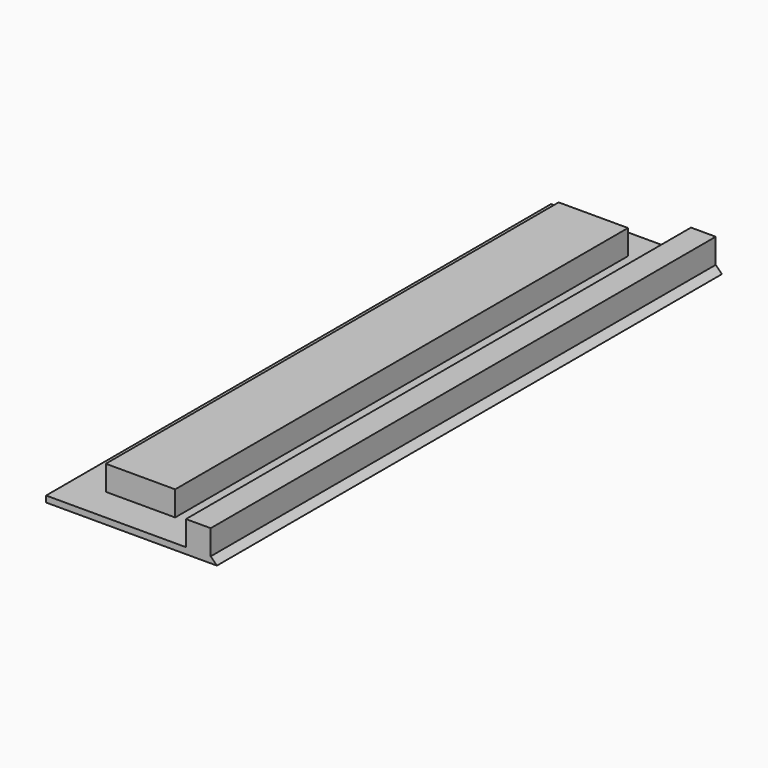
from build123d import *

# Parameters (mm, degrees)
F0_W     = 69
F0_H     = 255
F1_DEPTH = 2.5
F2_SIZE  = 2.49999
F3_W     = 10
F3_H     = 255
F4_DEPTH = 10
F5_W     = 28.0150985345
F5_H     = 228.639356792
F6_DEPTH = 10


# Not quite as in the source:
# - a fillet or chamfer is up to 0.001 mm smaller than in the source, because OpenCascade refuses the exact size


with BuildPart() as f1:
    # F0 (on Top) → F1 (new body)
    with BuildSketch(Plane.XY):
        Rectangle(F0_W, F0_H)
    extrude(amount=F1_DEPTH)

    # F2 (size 2.5 in the source; OpenCascade refuses exactly that, so slightly less here)
    f2_edges = [f1.edges().sort_by_distance(p)[0] for p in [
        (34.5, 0, 2.5),
    ]]
    chamfer(f2_edges, length=F2_SIZE)

    # F3 (on face) → F4 (join)
    with BuildSketch(Plane.XY.offset(2.5)):
        with Locations((27, 0)):
            Rectangle(F3_W, F3_H)
    extrude(amount=F4_DEPTH)

    # F5 (on face) → F6 (join)
    with BuildSketch(Plane.XY.offset(2.5)):
        with Locations((-7.3420391418, 0.5451031029)):
            Rectangle(F5_W, F5_H)
    extrude(amount=F6_DEPTH)


solid = f1.part
